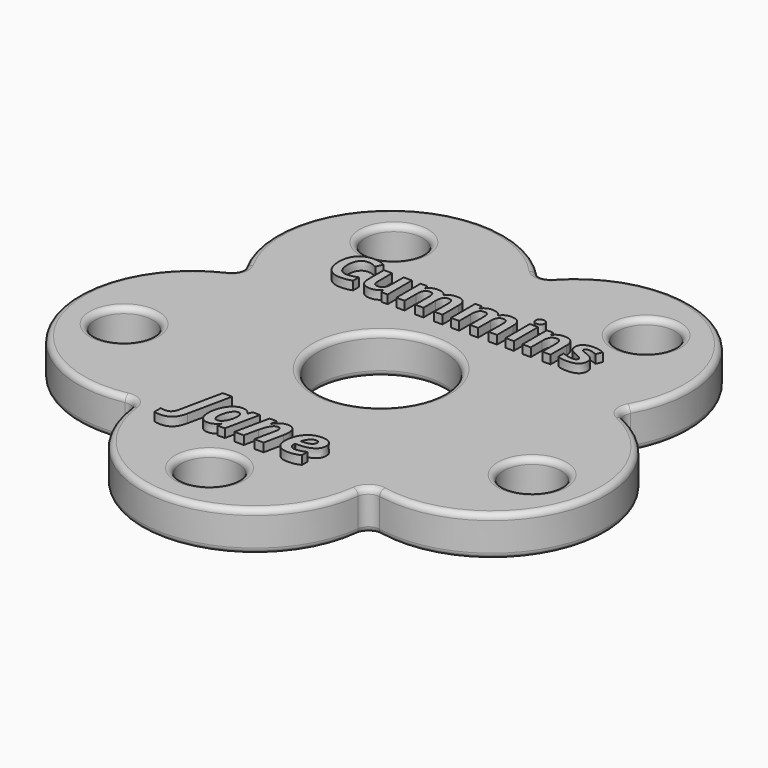
from build123d import *

# Parameters (mm, degrees)
F0_R           = 5
F0_R_2         = 11
F1_DEPTH       = 7
F2_R           = 2
F3_R           = 1
F4_TEXT_SIZE   = 11.1111111111
F4_TEXT_SIZE_2 = 9.7222222222
F5_DEPTH       = 1.5


# Not quite as in the source:
# - Text() gives the source's letters only with a copy of the font that has no kerning and outlines rounded to 1/6400 em; it was checked with that copy


with BuildPart() as f1:
    # F0 (on Top) → F1 (new body)
    with BuildSketch(Plane.XY):
        with BuildLine():
            ThreePointArc((32.360648934, 10.5146122215), (27.9197994839, 38.4283072328), (0, 34.0259999059))
            ThreePointArc((0, 34.0259999059), (-27.9197994839, 38.4283072328), (-32.360648934, 10.5146122215))
            ThreePointArc((-32.360648934, 10.5146122215), (-45.175184524, -14.6783072328), (-19.9999809392, -27.5276121745))
            ThreePointArc((-19.9999809392, -27.5276121745), (0, -47.5), (19.9999809392, -27.5276121745))
            ThreePointArc((19.9999809392, -27.5276121745), (45.175184524, -14.6783072328), (32.360648934, 10.5146122215))
        make_face()
        with Locations((-35.6646193611, -11.5881372891)):
            Circle(F0_R, mode=Mode.SUBTRACT)
        with Locations((0, -37.5)):
            Circle(F0_R, mode=Mode.SUBTRACT)
        with Locations((35.6646193611, -11.5881372891)):
            Circle(F0_R, mode=Mode.SUBTRACT)
        with Locations((-22.041946961, 30.3381372891)):
            Circle(F0_R, mode=Mode.SUBTRACT)
        Circle(F0_R_2, mode=Mode.SUBTRACT)
        with Locations((22.041946961, 30.3381372891)):
            Circle(F0_R, mode=Mode.SUBTRACT)
    extrude(amount=F1_DEPTH)

    # F2
    f2_edges = [f1.edges().sort_by_distance(p)[0] for p in [
        (19.999981, -27.527612, 3.5),
        (32.360649, 10.514612, 3.5),
        (0, 34.026, 3.5),
        (-32.360649, 10.514612, 3.5),
        (-19.999981, -27.527612, 3.5),
    ]]
    fillet(f2_edges, radius=F2_R)

    # F3
    f3_edges = [f1.edges().sort_by_distance(p)[0] for p in [
        (27.919799, 38.428307, 7),
        (33.45041, 10.868697, 7),
        (0, 35.171843, 7),
        (45.175185, -14.678307, 7),
        (-27.919799, 38.428307, 7),
        (20.67349, -28.454618, 7),
        (-33.45041, 10.868697, 7),
        (0, -47.5, 7),
        (-45.175185, -14.678307, 7),
        (-20.67349, -28.454618, 7),
        (-40.664619, -11.588137, 7),
        (-5, -37.5, 7),
        (30.664619, -11.588137, 7),
        (-27.041947, 30.338137, 7),
        (-11, 0, 7),
        (17.041947, 30.338137, 7),
        (27.919799, 38.428307, 0),
        (33.45041, 10.868697, 0),
        (0, 35.171843, 0),
        (45.175185, -14.678307, 0),
        (-27.919799, 38.428307, 0),
        (20.67349, -28.454618, 0),
        (-33.45041, 10.868697, 0),
        (0, -47.5, 0),
        (-45.175185, -14.678307, 0),
        (-20.67349, -28.454618, 0),
        (-40.664619, -11.588137, 0),
        (-5, -37.5, 0),
        (30.664619, -11.588137, 0),
        (-27.041947, 30.338137, 0),
        (-11, 0, 0),
        (17.041947, 30.338137, 0),
    ]]
    fillet(f3_edges, radius=F3_R)

    # F4 (on face) → F5 (join)
    with BuildSketch(Plane.XY.offset(7)):
        with Locations((-12.6866319444, -29.2949217986)):
            Text('Jane', F4_TEXT_SIZE, font='Open Sans', font_style=FontStyle.BOLDITALIC, text_align=(TextAlign.LEFT, TextAlign.BOTTOM))
        with Locations((-23.0629340278, 15.4673896549)):
            Text('Cummins', F4_TEXT_SIZE_2, font='Open Sans', font_style=FontStyle.BOLD, text_align=(TextAlign.LEFT, TextAlign.BOTTOM))
    extrude(amount=F5_DEPTH)


solid = f1.part
